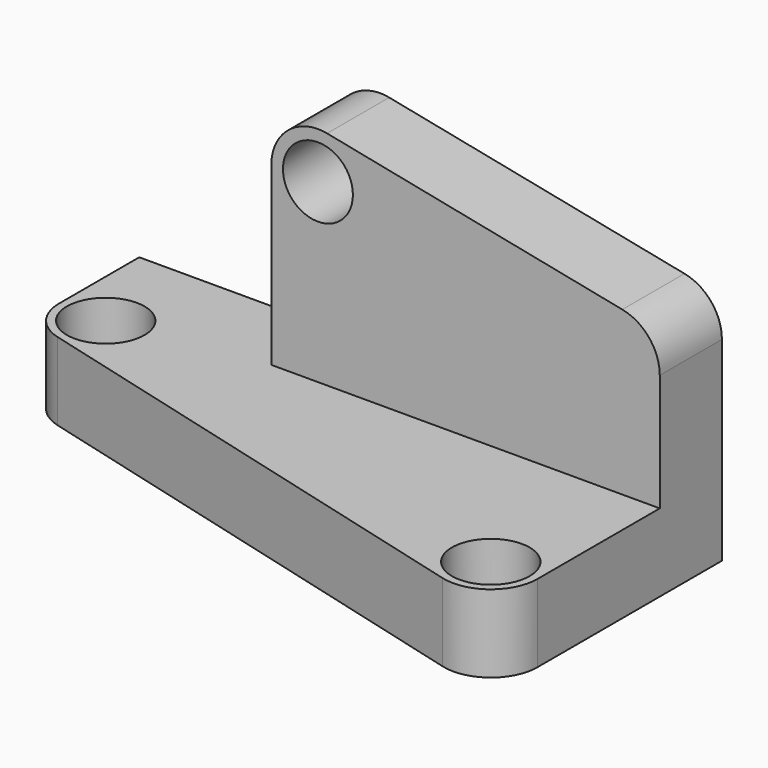
from build123d import *

# Parameters (mm, degrees)
F1_DEPTH  = 20
F3_DEPTH  = 20
F4_R      = 12
F5_R      = 10
F6_DEPTH  = 25
F7_R      = 10
F8_DEPTH  = 25
F9_R      = 9
F10_DEPTH = 25


with BuildPart() as f1:
    # F0 (on Top) → F1 (new body)
    with BuildSketch(Plane.XY):
        Polygon((150, 0), (0, 0), (0, -35), (150, -75), align=None)
    extrude(amount=-F1_DEPTH)

    # F2 (on face) → F3 (join)
    with BuildSketch(Plane(origin=(0, 0, 0), x_dir=(-1, 0, 0), z_dir=(0, 1, 0))):
        Polygon((-150, 40), (-150, 0), (-50, 0), (-50, 60), align=None)
    extrude(amount=-F3_DEPTH)

    # F4
    f4_edges = [f1.edges().sort_by_distance(p)[0] for p in [
        (0, -35, -10),
        (150, -75, -10),
        (50, -10, 60),
        (150, -10, 40),
    ]]
    fillet(f4_edges, radius=F4_R)

    # F5 (on face) → F6 (cut)
    with BuildSketch(Plane.XY):
        with Locations((12, -25.780660243)):
            Circle(F5_R)
    extrude(amount=-F6_DEPTH, mode=Mode.SUBTRACT)

    # F7 (on face) → F8 (cut)
    with BuildSketch(Plane.XY):
        with Locations((138, -59.380660243)):
            Circle(F7_R)
    extrude(amount=-F8_DEPTH, mode=Mode.SUBTRACT)

    # F9 (on face) → F10 (cut)
    with BuildSketch(Plane.XZ.offset(20)):
        with Locations((62, 45.3623531674)):
            Circle(F9_R)
    extrude(amount=-F10_DEPTH, mode=Mode.SUBTRACT)


solid = f1.part
